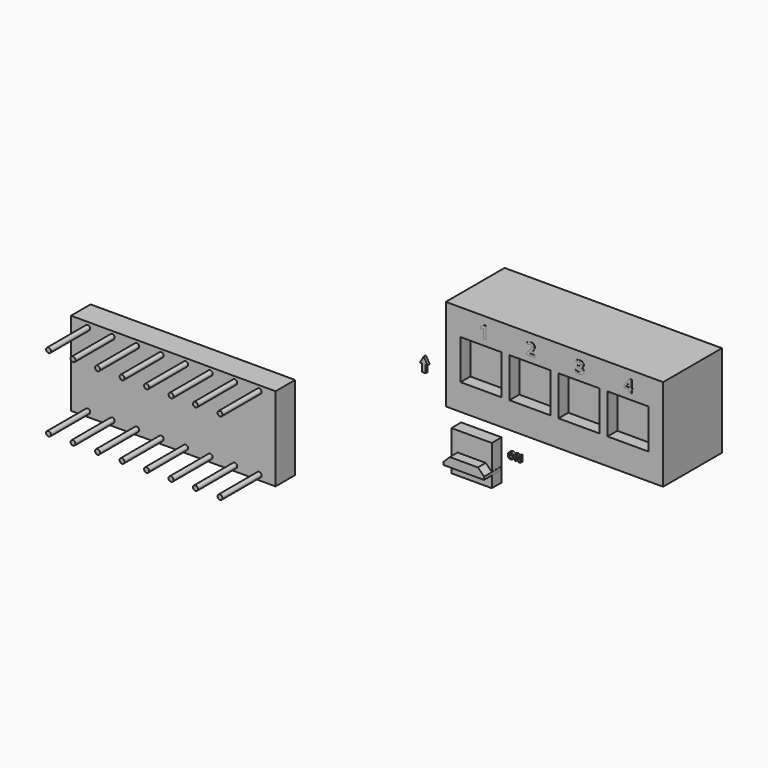
from build123d import *

# Parameters (mm, degrees)
F0_W          = 22.5298
F0_H          = 9.5504
F1_DEPTH      = 7.62
F2_W          = 4.2418
F2_H          = 4.1148
F3_DEPTH      = 1.27
F4_W          = 4.1857082397
F4_H          = 4.1301457677
F5_DEPTH      = 1.27
F6_W          = 4.1833990254
F6_H          = 0.9382874705
F7_DEPTH      = 2.286
F8_SIZE       = 0.635
F9_W          = 21.2126933038
F9_H          = 8.6868
F10_DEPTH     = 2.54
F11_R         = 0.254
F12_DEPTH     = 5.08
F13_TEXT_SIZE = 1.7638888889
F14_DEPTH     = 0.0254
F15_TEXT_SIZE = 0.8819444444
F16_DEPTH     = 0.2794
F17_W         = 0.3809110595
F17_H         = 0.7890465192
F18_DEPTH     = 0.2794


# Not quite as in the source:
# - Text() gives the source's letters only with a copy of the font that has no kerning and outlines rounded to 1/6400 em; it was checked with that copy


with BuildPart() as f1:
    # F0 (on Front) → F1 (new body)
    with BuildSketch(Plane.XZ):
        with Locations((0.2870801836, 0.0095496721)):
            Rectangle(F0_W, F0_H)
    extrude(amount=-F1_DEPTH)

    # F2 (on Front) → F3 (cut)
    with BuildSketch(Plane.XZ):
        with Locations((-7.3329198164, 0.0095496721)):
            Rectangle(F2_W, F2_H)
        with Locations((-2.2529198164, 0.0095496721)):
            Rectangle(F2_W, F2_H)
        with Locations((2.8270801836, 0.0095496721)):
            Rectangle(F2_W, F2_H)
        with Locations((7.9070801836, 0.0095496721)):
            Rectangle(F2_W, F2_H)
    extrude(amount=-F3_DEPTH, mode=Mode.SUBTRACT)


with BuildPart() as f5:
    # F4 (on Front) → F5 (new body)
    with BuildSketch(Plane.XZ):
        with Locations((-7.289560046, -7.7652913751)):
            Rectangle(F4_W, F4_H)
    extrude(amount=F5_DEPTH)


with BuildPart() as f7:
    # F6 (on Front) → F7 (new body)
    with BuildSketch(Plane.XZ):
        with Locations((-7.2814456653, -8.1908076536)):
            Rectangle(F6_W, F6_H)
    extrude(amount=F7_DEPTH)

    # F8
    f8_edges = [f7.edges().sort_by_distance(p)[0] for p in [
        (-5.189746, -1.143, -7.721664),
        (-9.373145, -1.143, -7.721664),
    ]]
    chamfer(f8_edges, length=F8_SIZE)


with BuildPart() as f10:
    # F9 (on Front) → F10 (new body)
    with BuildSketch(Plane.XZ):
        with Locations((-39.2355974764, -13.4594405427)):
            Rectangle(F9_W, F9_H)
    extrude(amount=-F10_DEPTH)


with BuildPart() as f12:
    # F11 (on Front) → F12 (new body)
    with BuildSketch(Plane.XZ):
        with Locations((-32.8649058938, -9.6494405427)):
            Circle(F11_R)
    extrude(amount=F12_DEPTH)


with BuildPart() as f12b:
    # F11 (on Front) → F12, piece 2 (new body)
    with BuildSketch(Plane.XZ):
        with Locations((-35.403970629, -9.6494405427)):
            Circle(F11_R)
    extrude(amount=F12_DEPTH)


with BuildPart() as f12c:
    # F11 (on Front) → F12, piece 3 (new body)
    with BuildSketch(Plane.XZ):
        with Locations((-37.9452556372, -9.6494405427)):
            Circle(F11_R)
    extrude(amount=F12_DEPTH)


with BuildPart() as f12d:
    # F11 (on Front) → F12, piece 4 (new body)
    with BuildSketch(Plane.XZ):
        with Locations((-40.485098958, -9.6494405427)):
            Circle(F11_R)
    extrude(amount=F12_DEPTH)


with BuildPart() as f12e:
    # F11 (on Front) → F12, piece 5 (new body)
    with BuildSketch(Plane.XZ):
        with Locations((-43.02559793, -9.6494405427)):
            Circle(F11_R)
    extrude(amount=F12_DEPTH)


with BuildPart() as f12f:
    # F11 (on Front) → F12, piece 6 (new body)
    with BuildSketch(Plane.XZ):
        with Locations((-45.5655306578, -9.6494405427)):
            Circle(F11_R)
    extrude(amount=F12_DEPTH)


with BuildPart() as f12g:
    # F11 (on Front) → F12, piece 7 (new body)
    with BuildSketch(Plane.XZ):
        with Locations((-48.1052175164, -9.6494405427)):
            Circle(F11_R)
    extrude(amount=F12_DEPTH)


with BuildPart() as f12h:
    # F11 (on Front) → F12, piece 8 (new body)
    with BuildSketch(Plane.XZ):
        with Locations((-48.105224967, -17.2694405427)):
            Circle(F11_R)
    extrude(amount=F12_DEPTH)


with BuildPart() as f12i:
    # F11 (on Front) → F12, piece 9 (new body)
    with BuildSketch(Plane.XZ):
        with Locations((-45.5651730299, -17.2694405427)):
            Circle(F11_R)
    extrude(amount=F12_DEPTH)


with BuildPart() as f12j:
    # F11 (on Front) → F12, piece 10 (new body)
    with BuildSketch(Plane.XZ):
        with Locations((-43.0252254009, -17.2694405427)):
            Circle(F11_R)
    extrude(amount=F12_DEPTH)


with BuildPart() as f12k:
    # F11 (on Front) → F12, piece 11 (new body)
    with BuildSketch(Plane.XZ):
        with Locations((-40.485162288, -17.2694405427)):
            Circle(F11_R)
    extrude(amount=F12_DEPTH)


with BuildPart() as f12l:
    # F11 (on Front) → F12, piece 12 (new body)
    with BuildSketch(Plane.XZ):
        with Locations((-37.9452109337, -17.2694405427)):
            Circle(F11_R)
    extrude(amount=F12_DEPTH)


with BuildPart() as f12m:
    # F11 (on Front) → F12, piece 13 (new body)
    with BuildSketch(Plane.XZ):
        with Locations((-35.4054197669, -17.2694405427)):
            Circle(F11_R)
    extrude(amount=F12_DEPTH)


with BuildPart() as f12n:
    # F11 (on Front) → F12, piece 14 (new body)
    with BuildSketch(Plane.XZ):
        with Locations((-32.8652560711, -17.2694405427)):
            Circle(F11_R)
    extrude(amount=F12_DEPTH)


with BuildPart() as f12o:
    # F11 (on Front) → F12, piece 15 (new body)
    with BuildSketch(Plane.XZ):
        with Locations((-30.3251743317, -17.2694405427)):
            Circle(F11_R)
    extrude(amount=F12_DEPTH)


with BuildPart() as f12p:
    # F11 (on Front) → F12, piece 16 (new body)
    with BuildSketch(Plane.XZ):
        with Locations((-30.3251035511, -9.6494405427)):
            Circle(F11_R)
    extrude(amount=F12_DEPTH)


with BuildPart() as f14:
    # F13 (on Front) → F14 (new body)
    with BuildSketch(Plane.XZ):
        with Locations((-7.5155264136, 2.7019496721)):
            Text('1', F13_TEXT_SIZE, font='Open Sans', font_style=FontStyle.BOLD, text_align=(TextAlign.LEFT, TextAlign.BOTTOM))
        with Locations((-2.6576661705, 2.7019496721)):
            Text('2', F13_TEXT_SIZE, font='Open Sans', font_style=FontStyle.BOLD, text_align=(TextAlign.LEFT, TextAlign.BOTTOM))
        with Locations((2.4344605656, 2.7019496721)):
            Text('3', F13_TEXT_SIZE, font='Open Sans', font_style=FontStyle.BOLD, text_align=(TextAlign.LEFT, TextAlign.BOTTOM))
        with Locations((7.4739462427, 2.7019496721)):
            Text('4', F13_TEXT_SIZE, font='Open Sans', font_style=FontStyle.BOLD, text_align=(TextAlign.LEFT, TextAlign.BOTTOM))
    extrude(amount=F14_DEPTH)


with BuildPart() as f16:
    # F15 (on Front) → F16 (new body)
    with BuildSketch(Plane.XZ):
        with Locations((-4.3692604374, -7.2148568229)):
            Text('ON', F15_TEXT_SIZE, font='Open Sans', font_style=FontStyle.BOLD, text_align=(TextAlign.LEFT, TextAlign.BOTTOM))
    extrude(amount=F16_DEPTH)


with BuildPart() as f18:
    # F17 (on Front) → F18 (new body)
    with BuildSketch(Plane.XZ):
        Polygon((-12.6510180729, -1.4423141267), (-13.0446736026, -0.7604827485), (-13.4383291324, -1.4423141267), (-13.2351291324, -1.4423141267), (-12.8542180729, -1.4423141267), align=None)
        with Locations((-13.0446736026, -1.8368373863)):
            Rectangle(F17_W, F17_H)
    extrude(amount=F18_DEPTH)


solid = Compound([f1.part, f5.part, f7.part, f10.part, f12.part, f12b.part, f12c.part, f12d.part, f12e.part, f12f.part, f12g.part, f12h.part, f12i.part, f12j.part, f12k.part, f12l.part, f12m.part, f12n.part, f12o.part, f12p.part, f14.part, f16.part, f18.part])
